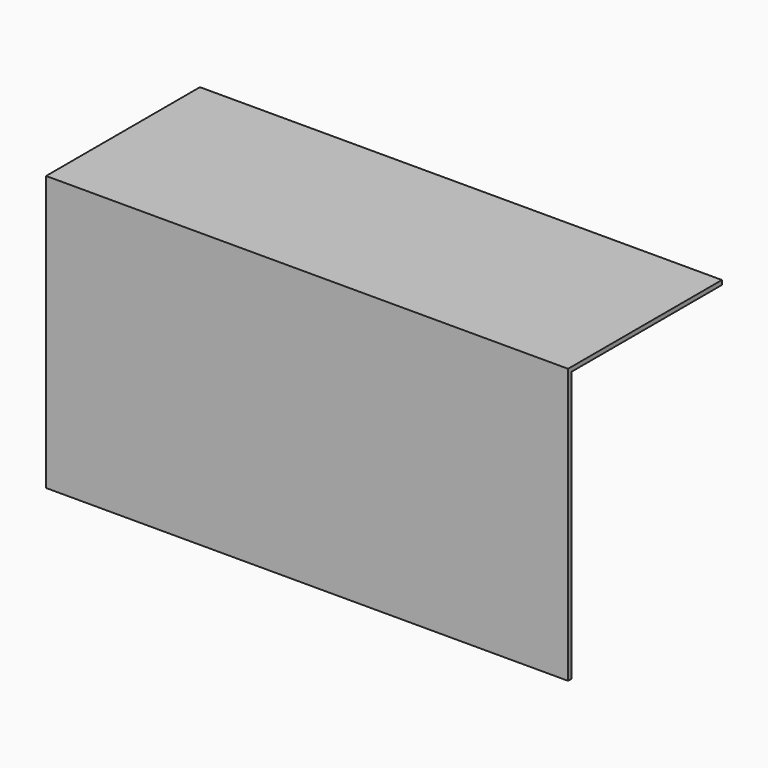
from build123d import *

# Parameters (mm, degrees)
F0_W     = 1900
F0_H     = 700
F1_DEPTH = 1000
F2_T     = -16


# Not quite as in the source:
# - a feature names something its author has since deleted; it is built from what else it names


with BuildPart() as f1:
    # F0 (on Top) → F1 (new body)
    with BuildSketch(Plane.XY):
        with Locations((-950, -350)):
            Rectangle(F0_W, F0_H)
    extrude(amount=F1_DEPTH)

    # F2
    f2_openings = [f1.faces().sort_by_distance(p)[0] for p in [
        (-950, -350, 0),
        (0, -350, 500),
        (-950, 0, 500),
    ]]
    offset(amount=F2_T, openings=f2_openings)


solid = f1.part
